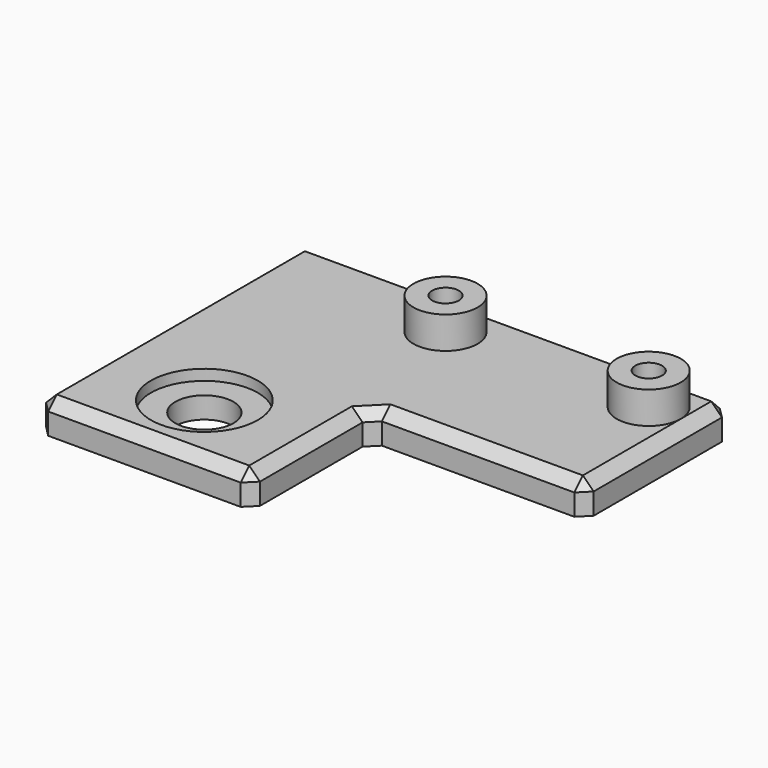
from build123d import *

# Parameters (mm, degrees)
F0_W     = 20
F0_H     = 14
F0_R     = 2.7148316461
F0_R_2   = 3
F0_R_3   = 1.25
F1_DEPTH = 3
F2_R     = 5
F2_R_2   = 2.7148316461
F3_DEPTH = 1
F4_DEPTH = 3
F5_SIZE  = 0.99999


# Not quite as in the source:
# - a fillet or chamfer is up to 0.001 mm smaller than in the source, because OpenCascade refuses the exact size


with BuildPart() as f1:
    # F0 (on Top) → F1 (new body)
    with BuildSketch(Plane.XY):
        with Locations((10, -7)):
            Rectangle(F0_W, F0_H)
        with Locations((10, -7)):
            Circle(F0_R, mode=Mode.SUBTRACT)
        Polygon((0, 17), (0, 0), (20, 0), (40, 0), (40, 17), align=None)
        with Locations((17, 12.44318299)):
            Circle(F0_R_2, mode=Mode.SUBTRACT)
        with Locations((36, 12.44318299)):
            Circle(F0_R_2, mode=Mode.SUBTRACT)
        with Locations((36, 12.44318299)):
            Circle(F0_R_2)
        with Locations((36, 12.44318299)):
            Circle(F0_R_3, mode=Mode.SUBTRACT)
        with Locations((17, 12.44318299)):
            Circle(F0_R_2)
        with Locations((17, 12.44318299)):
            Circle(F0_R_3, mode=Mode.SUBTRACT)
    extrude(amount=-F1_DEPTH)

    # F2 (on face) → F3 (cut)
    with BuildSketch(Plane.XY):
        with Locations((10, -7)):
            Circle(F2_R)
        with Locations((10, -7)):
            Circle(F2_R_2, mode=Mode.SUBTRACT)
    extrude(amount=-F3_DEPTH, mode=Mode.SUBTRACT)

    # F0 (on Top) → F4 (join)
    with BuildSketch(Plane.XY):
        with Locations((17, 12.44318299)):
            Circle(F0_R_2)
        with Locations((17, 12.44318299)):
            Circle(F0_R_3, mode=Mode.SUBTRACT)
        with Locations((36, 12.44318299)):
            Circle(F0_R_2)
        with Locations((36, 12.44318299)):
            Circle(F0_R_3, mode=Mode.SUBTRACT)
    extrude(amount=F4_DEPTH)

    # F5 (size 1 in the source; OpenCascade refuses exactly that, so slightly less here)
    f5_edges = [f1.edges().sort_by_distance(p)[0] for p in [
        (0, 1.5, 0),
        (10, -14, 0),
        (20, -7, 0),
        (30, 0, 0),
        (40, 8.5, 0),
        (20, 17, 0),
        (40, 0, -1.5),
        (40, 17, -1.5),
        (20, -14, -1.5),
        (0, 17, -1.5),
        (0, -14, -1.5),
        (20, 0, -1.5),
    ]]
    chamfer(f5_edges, length=F5_SIZE)


solid = f1.part
